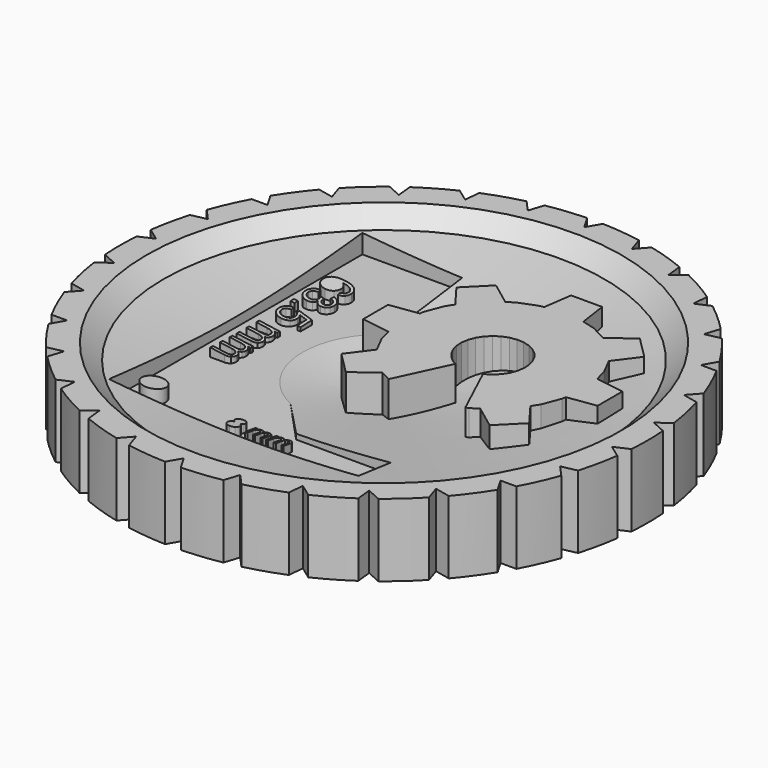
from build123d import *

# Parameters (mm, degrees)
F4_DEPTH        = 64
F4_COPIES_COUNT = 30
F5_R            = 1.080516378
F5_W            = 0.3783217323
F5_H            = 0.3783222047
F6_DEPTH        = 28.3


# Not quite as in the source:
# - ends of sketch curves that miss each other by under 0.0002 mm in the source are joined
# - the dataset's text gives a spline's control points without its knots; the knots are read off the source's solid
# - a pattern or mirror of a feature is missing from the dataset's text; its kind, count and spacing are read off the source's solid


with BuildPart() as f1:
    # F0 (on Front) → F1 (revolve)
    with BuildSketch(Plane.XZ):
        Polygon((-25, 0), (0, 0), (0, 2.5), (-20.8576644046, 5.4197078553), (-22.5, 6.8795619782), (-25, 6.8795619782), align=None)
    revolve(axis=Axis((0, 0, 1.25), (0, 0, -1)))

    # F3 (on offset) → F4 (cut)
    with BuildSketch(Plane.XY.offset(31.8795619782)):
        Polygon((1.4257947543, 26.1719338596), (-1.4257947543, 26.1719338596), (0, 23.702384904), align=None)
    f4 = extrude(amount=-F4_DEPTH, mode=Mode.SUBTRACT)

    # F4_copies: F4 ×30 about axis
    f4_copies_axis = Axis((0, 0, 0), (0, 0, 1))
    for i in range(1, F4_COPIES_COUNT):
        add(f4.rotate(f4_copies_axis, i * 360 / F4_COPIES_COUNT), mode=Mode.SUBTRACT)

    # F5 (on offset) → F6 (cut)
    with BuildSketch(Plane.XY.offset(31.8795619782)):
        Polygon((-14.0490727499, 14.9999975413), (-14.0490727499, -15.0000024587), (9.5729744942, -15.0000024587), (9.5990074076, -11.2204748996), (0.659531817, -11.2204748996), (-4.6002538523, -5.5511835611), (-4.6002538523, 14.9999975413), align=None)
        with Locations((-11.6868680255, -12.6377977343)):
            Circle(F5_R, mode=Mode.SUBTRACT)
        with BuildLine():
            add(Edge.make_bspline(
                [(-3.9348817263, -13.1844435611), (-3.9031511751, -13.150072065), (-3.8372267657, -13.0786621437), (-3.7446949546, -13.0484429311), (-3.6967006239, -13.0327687579)],
                knots=[0, 0, 0, 0, 0.291983, 0.606627, 0.606627, 0.606627, 0.606627], degree=3))
            add(Edge.make_bspline(
                [(-3.6967006239, -13.0327687579), (-3.7361725924, -13.016399624), (-3.8102612538, -12.9856748996), (-3.8633593641, -12.9257958445), (-3.888168183, -12.8978183642)],
                knots=[0, 0, 0, 0, 0.267234, 0.501594, 0.501594, 0.501594, 0.501594], degree=3))
            add(Edge.make_bspline(
                [(-3.888168183, -12.8978183642), (-3.9063288129, -12.8664988366), (-3.9439445609, -12.8016256083), (-3.9482343247, -12.7266662382), (-3.9504529074, -12.6878958445)],
                knots=[0, 0, 0, 0, 0.226571, 0.469298, 0.469298, 0.469298, 0.469298], degree=3))
            add(Edge.make_bspline(
                [(-3.9504529074, -12.6878958445), (-3.9449877105, -12.6288893878), (-3.9340866082, -12.5112010414), (-3.8564971594, -12.4220689154), (-3.8178099153, -12.3776259233)],
                knots=[0, 0, 0, 0, 0.366285, 0.730555, 0.730555, 0.730555, 0.730555], degree=3))
            add(Edge.make_bspline(
                [(-3.8178099153, -12.3776259233), (-3.7682073956, -12.3409834036), (-3.6635744822, -12.2636892303), (-3.533351805, -12.2559652933), (-3.4648629861, -12.2519032461)],
                knots=[0, 0, 0, 0, 0.383224, 0.808383, 0.808383, 0.808383, 0.808383], degree=3))
            add(Edge.make_bspline(
                [(-3.4648629861, -12.2519032461), (-3.3958516476, -12.2561580492), (-3.2641351121, -12.2642783642), (-3.1586659783, -12.3430229311), (-3.108456372, -12.3805097028)],
                knots=[0, 0, 0, 0, 0.428413, 0.817672, 0.817672, 0.817672, 0.817672], degree=3))
            add(Edge.make_bspline(
                [(-3.108456372, -12.3805097028), (-3.0690958995, -12.4256211988), (-2.9905988916, -12.5155876555), (-2.9791927499, -12.6344174193), (-2.9735059783, -12.6936629311)],
                knots=[0, 0, 0, 0, 0.370122, 0.73814, 0.73814, 0.73814, 0.73814], degree=3))
            add(Edge.make_bspline(
                [(-2.9735059783, -12.6936629311), (-2.9757977893, -12.7312045059), (-2.980264246, -12.8043752146), (-3.0172195216, -12.8676057658), (-3.0352143247, -12.8983952146)],
                knots=[0, 0, 0, 0, 0.235128, 0.45828, 0.45828, 0.45828, 0.45828], degree=3))
            add(Edge.make_bspline(
                [(-3.0352143247, -12.8983952146), (-3.0596026712, -12.9261794666), (-3.111556057, -12.9853659233), (-3.1841362145, -13.0163367894), (-3.2226448759, -13.0327687579)],
                knots=[0, 0, 0, 0, 0.231762, 0.493704, 0.493704, 0.493704, 0.493704], degree=3))
            add(Edge.make_bspline(
                [(-3.2226448759, -13.0327687579), (-3.1744984192, -13.0513942697), (-3.0822292853, -13.0870886004), (-3.0168708601, -13.1611423012), (-2.9856170019, -13.1965545847)],
                knots=[0, 0, 0, 0, 0.322391, 0.617832, 0.617832, 0.617832, 0.617832], degree=3))
            add(Edge.make_bspline(
                [(-2.9856170019, -13.1965545847), (-2.9619066082, -13.2368476555), (-2.9129177893, -13.3200983642), (-2.9072338523, -13.4166393091), (-2.9043009389, -13.4664548996)],
                knots=[0, 0, 0, 0, 0.29248, 0.604301, 0.604301, 0.604301, 0.604301], degree=3))
            add(Edge.make_bspline(
                [(-2.9043009389, -13.4664548996), (-2.9105593641, -13.5357232461), (-2.923012435, -13.6735479705), (-3.0129628287, -13.7786542697), (-3.0577058208, -13.8309355296)],
                knots=[0, 0, 0, 0, 0.430093, 0.855761, 0.855761, 0.855761, 0.855761], degree=3))
            add(Edge.make_bspline(
                [(-3.0577058208, -13.8309355296), (-3.1146108601, -13.8739725374), (-3.2337902302, -13.9641076555), (-3.3832870806, -13.9736089154), (-3.4614028287, -13.9785733248)],
                knots=[0, 0, 0, 0, 0.443046, 0.927898, 0.927898, 0.927898, 0.927898], degree=3))
            add(Edge.make_bspline(
                [(-3.4614028287, -13.9785733248), (-3.5395341672, -13.9735753721), (-3.6891316476, -13.9640060807), (-3.8082127499, -13.8735643485), (-3.8650998365, -13.8303586792)],
                knots=[0, 0, 0, 0, 0.484901, 0.928432, 0.928432, 0.928432, 0.928432], degree=3))
            add(Edge.make_bspline(
                [(-3.8650998365, -13.8303586792), (-3.9098418838, -13.7775189941), (-4.0002821987, -13.6707095453), (-4.0123880255, -13.5311868681), (-4.0185047184, -13.460687813)],
                knots=[0, 0, 0, 0, 0.428425, 0.866013, 0.866013, 0.866013, 0.866013], degree=3))
            add(Edge.make_bspline(
                [(-4.0185047184, -13.460687813), (-4.0157031436, -13.4088813563), (-4.0103451909, -13.3097972618), (-3.9592582617, -13.2249355296), (-3.9348817263, -13.1844435611)],
                knots=[0, 0, 0, 0, 0.323778, 0.619255, 0.619255, 0.619255, 0.619255], degree=3))
        make_face(mode=Mode.SUBTRACT)
        with BuildLine():
            Line((-12.5727103877, -2.550036002), (-12.5727103877, -2.2178509626))
            Line((-12.5727103877, -2.2178509626), (-10.6128188916, -2.2178509626))
            Line((-10.6128188916, -2.2178509626), (-10.6128188916, -2.5149714351))
            Line((-10.6128188916, -2.5149714351), (-10.8877941672, -2.5149714351))
            add(Edge.make_bspline(
                [(-10.8877941672, -2.5149714351), (-10.8420387342, -2.5484750571), (-10.7497648759, -2.6160407264), (-10.6875514901, -2.7120293878), (-10.6561875531, -2.7604205689)],
                knots=[0, 0, 0, 0, 0.356855, 0.719659, 0.719659, 0.719659, 0.719659], degree=3))
            add(Edge.make_bspline(
                [(-10.6561875531, -2.7604205689), (-10.6306251909, -2.8140846634), (-10.5780789601, -2.9243975906), (-10.5717685144, -3.0465068651), (-10.5685275777, -3.1092133202)],
                knots=[0, 0, 0, 0, 0.373568, 0.767905, 0.767905, 0.767905, 0.767905], degree=3))
            add(Edge.make_bspline(
                [(-10.5685275777, -3.1092133202), (-10.5710919625, -3.1765810414), (-10.5758792066, -3.3023174193), (-10.6326165294, -3.414319939), (-10.6589555846, -3.4663134823)],
                knots=[0, 0, 0, 0, 0.422154, 0.787929, 0.787929, 0.787929, 0.787929], degree=3))
            add(Edge.make_bspline(
                [(-10.6589555846, -3.4663134823), (-10.6923566869, -3.5094260807), (-10.7598154864, -3.5964996549), (-10.8608004877, -3.6405935115), (-10.9117847502, -3.6628553372)],
                knots=[0, 0, 0, 0, 0.340443, 0.687583, 0.687583, 0.687583, 0.687583], degree=3))
            add(Edge.make_bspline(
                [(-10.9117847502, -3.6628553372), (-10.8116985767, -3.7441177343), (-10.6176892853, -3.9016366319), (-10.5845640885, -4.1486093878), (-10.5685275531, -4.2681714351)],
                knots=[0, 0, 0, 0, 0.785976, 1.523536, 1.523536, 1.523536, 1.523536], degree=3))
            add(Edge.make_bspline(
                [(-10.5685275531, -4.2681714351), (-10.5730776318, -4.357499624), (-10.5815631436, -4.5240865532), (-10.6829740098, -4.6556193091), (-10.7300064507, -4.7166213563)],
                knots=[0, 0, 0, 0, 0.552547, 1.030438, 1.030438, 1.030438, 1.030438], degree=3))
            add(Edge.make_bspline(
                [(-10.7300064507, -4.7166213563), (-10.796196372, -4.7622308051), (-10.9449448759, -4.8647297028), (-11.1265606239, -4.8703607264), (-11.2273610964, -4.8734863957)],
                knots=[0, 0, 0, 0, 0.50044, 1.124636, 1.124636, 1.124636, 1.124636], degree=3))
            Line((-11.2273610964, -4.8734863957), (-12.5727103877, -4.8734863957))
            Line((-12.5727103877, -4.8734863957), (-12.5727103877, -4.5431462382))
            Line((-12.5727103877, -4.5431462382), (-11.3380894428, -4.5431462382))
            add(Edge.make_bspline(
                [(-11.3380894428, -4.5431462382), (-11.2806151121, -4.5431325374), (-11.1835884979, -4.5431098603), (-11.0894810964, -4.5201926949), (-11.0511184192, -4.5108506477)],
                knots=[0, 0, 0, 0, 0.363195, 0.613139, 0.613139, 0.613139, 0.613139], degree=3))
            add(Edge.make_bspline(
                [(-11.0511184192, -4.5108506477), (-11.0231555846, -4.4976279705), (-10.9661244035, -4.4706600965), (-10.9289088129, -4.4196586792), (-10.9099398365, -4.3936635611)],
                knots=[0, 0, 0, 0, 0.193139, 0.393917, 0.393917, 0.393917, 0.393917], degree=3))
            add(Edge.make_bspline(
                [(-10.9099398365, -4.3936635611), (-10.8943355846, -4.3635147422), (-10.8620038358, -4.3010471353), (-10.8583247684, -4.230732391), (-10.8564213289, -4.1943539714)],
                knots=[0, 0, 0, 0, 0.212991, 0.441316, 0.441316, 0.441316, 0.441316], degree=3))
            add(Edge.make_bspline(
                [(-10.8564213289, -4.1943539714), (-10.8617229861, -4.1288065532), (-10.8721384192, -4.0000474981), (-10.95381212, -3.9001418288), (-10.9939086554, -3.8510939548)],
                knots=[0, 0, 0, 0, 0.406947, 0.799408, 0.799408, 0.799408, 0.799408], degree=3))
            add(Edge.make_bspline(
                [(-10.9939086554, -3.8510939548), (-11.051635742, -3.8114150571), (-11.1832118301, -3.7209748331), (-11.343877466, -3.7168465615), (-11.4340535249, -3.7145297152)],
                knots=[0, 0, 0, 0, 0.436121, 0.994043, 0.994043, 0.994043, 0.994043], degree=3))
            Line((-11.4340535249, -3.7145297152), (-12.5727103877, -3.7145297028))
            Line((-12.5727103877, -3.7145297028), (-12.5727103877, -3.3823446634))
            Line((-12.5727103877, -3.3823446634), (-11.2993346397, -3.3823446634))
            add(Edge.make_bspline(
                [(-11.2993346397, -3.3823446634), (-11.2332944822, -3.381036002), (-11.1159987342, -3.3787115925), (-11.0124136948, -3.3247314351), (-10.9671496003, -3.3011434036)],
                knots=[0, 0, 0, 0, 0.412401, 0.732475, 0.732475, 0.732475, 0.732475], degree=3))
            add(Edge.make_bspline(
                [(-10.9671496003, -3.3011434036), (-10.9349173168, -3.2674758445), (-10.8643549546, -3.1937708051), (-10.8592138523, -3.0911434036), (-10.8564212538, -3.0353948996)],
                knots=[0, 0, 0, 0, 0.286757, 0.627767, 0.627767, 0.627767, 0.627767], degree=3))
            add(Edge.make_bspline(
                [(-10.8564212538, -3.0353948996), (-10.8594925924, -2.9895345847), (-10.8656329074, -2.8978470256), (-10.9087096003, -2.8166769469), (-10.9302401515, -2.7761065532)],
                knots=[0, 0, 0, 0, 0.288303, 0.576397, 0.576397, 0.576397, 0.576397], degree=3))
            add(Edge.make_bspline(
                [(-10.9302401515, -2.7761065532), (-10.9581902302, -2.7389741122), (-11.0153403701, -2.6630492008), (-11.1019220644, -2.623673615), (-11.1461598713, -2.6035552562)],
                knots=[0, 0, 0, 0, 0.290214, 0.593409, 0.593409, 0.593409, 0.593409], degree=3))
            add(Edge.make_bspline(
                [(-11.1461598713, -2.6035552562), (-11.2036776318, -2.5880235611), (-11.3376221987, -2.5518539548), (-11.476571805, -2.5506964744), (-11.5558549546, -2.550036002)],
                knots=[0, 0, 0, 0, 0.376888, 0.87769, 0.87769, 0.87769, 0.87769], degree=3))
            Line((-11.5558549546, -2.550036002), (-12.5727103877, -2.550036002))
        make_face(mode=Mode.SUBTRACT)
        with BuildLine():
            Line((-12.5727103877, 0.5983406909), (-12.5727103877, 0.9305257303))
            Line((-12.5727103877, 0.9305257303), (-10.6128188916, 0.9305257303))
            Line((-10.6128188916, 0.9305257303), (-10.6128188916, 0.633404313))
            Line((-10.6128188916, 0.633404313), (-10.8877941672, 0.633404313))
            add(Edge.make_bspline(
                [(-10.8877941672, 0.633404313), (-10.8420387342, 0.5999011634), (-10.7497648759, 0.5323354941), (-10.6875514901, 0.4363477775), (-10.6561875531, 0.3879570689)],
                knots=[0, 0, 0, 0, 0.356855, 0.719659, 0.719659, 0.719659, 0.719659], degree=3))
            add(Edge.make_bspline(
                [(-10.6561875531, 0.3879570689), (-10.6306251909, 0.3342920295), (-10.5780793641, 0.2239784862), (-10.5717684979, 0.1018690374), (-10.5685275531, 0.0391628956)],
                knots=[0, 0, 0, 0, 0.373568, 0.767906, 0.767906, 0.767906, 0.767906], degree=3))
            add(Edge.make_bspline(
                [(-10.5685275531, 0.0391628956), (-10.571092435, -0.028203876), (-10.5758792066, -0.153940254), (-10.6326165294, -0.2659427737), (-10.6589555846, -0.3179367894)],
                knots=[0, 0, 0, 0, 0.422154, 0.787929, 0.787929, 0.787929, 0.787929], degree=3))
            add(Edge.make_bspline(
                [(-10.6589555846, -0.3179367894), (-10.6923562145, -0.3610498603), (-10.7598151121, -0.4481245059), (-10.8608007814, -0.4922178918), (-10.9117851909, -0.5144788366)],
                knots=[0, 0, 0, 0, 0.340443, 0.687584, 0.687584, 0.687584, 0.687584], degree=3))
            add(Edge.make_bspline(
                [(-10.9117851909, -0.5144788366), (-10.8116985767, -0.5957415138), (-10.6176897578, -0.7532604114), (-10.5845640885, -1.0002331674), (-10.5685275531, -1.1197947422)],
                knots=[0, 0, 0, 0, 0.785976, 1.523536, 1.523536, 1.523536, 1.523536], degree=3))
            add(Edge.make_bspline(
                [(-10.5685275531, -1.1197947422), (-10.5730776318, -1.2091234036), (-10.5815626712, -1.3757108051), (-10.6829740098, -1.5072430886), (-10.7300064507, -1.5682446634)],
                knots=[0, 0, 0, 0, 0.552547, 1.030438, 1.030438, 1.030438, 1.030438], degree=3))
            add(Edge.make_bspline(
                [(-10.7300064507, -1.5682446634), (-10.796196372, -1.6138541122), (-10.9449448759, -1.7163530099), (-11.1265606239, -1.7219840335), (-11.2273610964, -1.7251097028)],
                knots=[0, 0, 0, 0, 0.50044, 1.124636, 1.124636, 1.124636, 1.124636], degree=3))
            Line((-11.2273610964, -1.7251097028), (-12.5727103877, -1.7251097028))
            Line((-12.5727103877, -1.7251097028), (-12.5727103877, -1.3947695453))
            Line((-12.5727103877, -1.3947695453), (-11.3380894428, -1.3947695453))
            add(Edge.make_bspline(
                [(-11.3380894428, -1.3947695453), (-11.2806151121, -1.3947558445), (-11.1835884979, -1.3947331674), (-11.0894810964, -1.371816002), (-11.0511184192, -1.3624739548)],
                knots=[0, 0, 0, 0, 0.363195, 0.613139, 0.613139, 0.613139, 0.613139], degree=3))
            add(Edge.make_bspline(
                [(-11.0511184192, -1.3624739548), (-11.0231555846, -1.3492512776), (-10.9661244035, -1.3222834036), (-10.9289088129, -1.2712819863), (-10.9099398365, -1.2452868681)],
                knots=[0, 0, 0, 0, 0.193139, 0.393917, 0.393917, 0.393917, 0.393917], degree=3))
            add(Edge.make_bspline(
                [(-10.9099398365, -1.2452868681), (-10.8943355846, -1.2151380492), (-10.8620031436, -1.1526704902), (-10.8583247184, -1.0823547422), (-10.8564212538, -1.0459748996)],
                knots=[0, 0, 0, 0, 0.212991, 0.441319, 0.441319, 0.441319, 0.441319], degree=3))
            add(Edge.make_bspline(
                [(-10.8564212538, -1.0459748996), (-10.8617229861, -0.9804289154), (-10.8721379468, -0.8516698603), (-10.95381212, -0.7517646634), (-10.9939086554, -0.7027172618)],
                knots=[0, 0, 0, 0, 0.406947, 0.799408, 0.799408, 0.799408, 0.799408], degree=3))
            add(Edge.make_bspline(
                [(-10.9939086554, -0.7027172618), (-11.051635742, -0.6630378918), (-11.1832114901, -0.5725966319), (-11.3438777893, -0.5684689154), (-11.4340540098, -0.566152065)],
                knots=[0, 0, 0, 0, 0.436121, 0.994044, 0.994044, 0.994044, 0.994044], degree=3))
            Line((-11.4340540098, -0.566152065), (-12.5727103877, -0.566152065))
            Line((-12.5727103877, -0.566152065), (-12.5727103877, -0.2339670256))
            Line((-12.5727103877, -0.2339670256), (-11.2993346397, -0.2339670256))
            add(Edge.make_bspline(
                [(-11.2993346397, -0.2339670256), (-11.2332944822, -0.2326588366), (-11.1159987342, -0.2303348996), (-11.0124136948, -0.1763547422), (-10.9671496003, -0.1527667107)],
                knots=[0, 0, 0, 0, 0.412401, 0.732475, 0.732475, 0.732475, 0.732475], degree=3))
            add(Edge.make_bspline(
                [(-10.9671496003, -0.1527667107), (-10.9349173168, -0.119099624), (-10.8643544822, -0.0453950571), (-10.8592138523, 0.0572328169), (-10.8564212538, 0.1129817933)],
                knots=[0, 0, 0, 0, 0.286757, 0.627767, 0.627767, 0.627767, 0.627767], degree=3))
            add(Edge.make_bspline(
                [(-10.8564212538, 0.1129817933), (-10.8594925924, 0.1588421082), (-10.8656329074, 0.2505296673), (-10.9087096003, 0.331699746), (-10.9302401515, 0.3722701397)],
                knots=[0, 0, 0, 0, 0.288303, 0.576397, 0.576397, 0.576397, 0.576397], degree=3))
            add(Edge.make_bspline(
                [(-10.9302401515, 0.3722701397), (-10.9581902302, 0.4094021082), (-11.0153404664, 0.48532762), (-11.1019223562, 0.5247032106), (-11.146160309, 0.5448221082)],
                knots=[0, 0, 0, 0, 0.290214, 0.59341, 0.59341, 0.59341, 0.59341], degree=3))
            add(Edge.make_bspline(
                [(-11.146160309, 0.5448221082), (-11.2036776318, 0.5603536043), (-11.3376221987, 0.5965232106), (-11.476571805, 0.5976802185), (-11.5558549546, 0.5983406909)],
                knots=[0, 0, 0, 0, 0.376888, 0.87769, 0.87769, 0.87769, 0.87769], degree=3))
            Line((-11.5558549546, 0.5983406909), (-12.5727103877, 0.5983406909))
        make_face(mode=Mode.SUBTRACT)
        with BuildLine():
            Line((-1.7808694428, -13.9497378918), (-1.9884850334, -13.9497378918))
            Line((-1.9884850334, -13.9497378918), (-1.9884850334, -12.7248052933))
            Line((-1.9884850334, -12.7248052933), (-1.8027845609, -12.7248052933))
            Line((-1.8027845609, -12.7248052933), (-1.8027845609, -12.8966651359))
            add(Edge.make_bspline(
                [(-1.8027845609, -12.8966651359), (-1.7818450334, -12.868067813), (-1.7396168444, -12.8103969469), (-1.679623931, -12.7715131674), (-1.649379679, -12.7519106477)],
                knots=[0, 0, 0, 0, 0.223034, 0.449787, 0.449787, 0.449787, 0.449787], degree=3))
            add(Edge.make_bspline(
                [(-1.649379679, -12.7519106477), (-1.6158392066, -12.7359345847), (-1.5468935373, -12.7030933248), (-1.4705749546, -12.6991489154), (-1.4313831436, -12.6971235611)],
                knots=[0, 0, 0, 0, 0.233479, 0.479942, 0.479942, 0.479942, 0.479942], degree=3))
            add(Edge.make_bspline(
                [(-1.4313831436, -12.6971235611), (-1.3892792066, -12.6987265532), (-1.3106938523, -12.7017180492), (-1.2406927499, -12.7371789941), (-1.208196372, -12.7536411988)],
                knots=[0, 0, 0, 0, 0.263846, 0.492455, 0.492455, 0.492455, 0.492455], degree=3))
            add(Edge.make_bspline(
                [(-1.208196372, -12.7536411988), (-1.1812507027, -12.7745164744), (-1.1268292853, -12.8166780492), (-1.0992708601, -12.8797942697), (-1.0853570019, -12.9116594666)],
                knots=[0, 0, 0, 0, 0.212777, 0.42974, 0.42974, 0.42974, 0.42974], degree=3))
            add(Edge.make_bspline(
                [(-1.0853570019, -12.9116594666), (-1.034568183, -12.8491049784), (-0.9361190491, -12.7278497028), (-0.7817617263, -12.7071459233), (-0.7070352696, -12.6971235611)],
                knots=[0, 0, 0, 0, 0.491234, 0.952209, 0.952209, 0.952209, 0.952209], degree=3))
            add(Edge.make_bspline(
                [(-0.7070352696, -12.6971235611), (-0.6512050334, -12.6999671831), (-0.5470880255, -12.7052703327), (-0.4648804664, -12.7686525374), (-0.4267540098, -12.798047813)],
                knots=[0, 0, 0, 0, 0.345341, 0.644024, 0.644024, 0.644024, 0.644024], degree=3))
            add(Edge.make_bspline(
                [(-0.4267540098, -12.798047813), (-0.398247868, -12.8394166319), (-0.3341862932, -12.9323845059), (-0.3306670806, -13.0458941122), (-0.3287135373, -13.1088945847)],
                knots=[0, 0, 0, 0, 0.312775, 0.702897, 0.702897, 0.702897, 0.702897], degree=3))
            Line((-0.3287135373, -13.1088945847), (-0.3287135373, -13.9497378918))
            Line((-0.3287135373, -13.9497378918), (-0.5351754271, -13.9497378918))
            Line((-0.5351754271, -13.9497378918), (-0.5351754271, -13.178099624))
            add(Edge.make_bspline(
                [(-0.5351754271, -13.178099624), (-0.535183931, -13.1421780492), (-0.5351985767, -13.0815364744), (-0.5495215688, -13.0227194666), (-0.5553604664, -12.9987426162)],
                knots=[0, 0, 0, 0, 0.226997, 0.383212, 0.383212, 0.383212, 0.383212], degree=3))
            add(Edge.make_bspline(
                [(-0.5553604664, -12.9987426162), (-0.5636244035, -12.9812660807), (-0.5804792066, -12.9456213563), (-0.6123552696, -12.9223616713), (-0.6286025137, -12.9105062382)],
                knots=[0, 0, 0, 0, 0.120712, 0.246199, 0.246199, 0.246199, 0.246199], degree=3))
            add(Edge.make_bspline(
                [(-0.6286025137, -12.9105062382), (-0.6474453483, -12.9007531674), (-0.686487868, -12.8805459233), (-0.7304347972, -12.8782465532), (-0.7531719625, -12.8770569469)],
                knots=[0, 0, 0, 0, 0.13312, 0.275823, 0.275823, 0.275823, 0.275823], degree=3))
            add(Edge.make_bspline(
                [(-0.7531719625, -12.8770569469), (-0.7941382617, -12.8803706477), (-0.8746129074, -12.886879939), (-0.9370535373, -12.9379262382), (-0.9677083405, -12.9629868681)],
                knots=[0, 0, 0, 0, 0.254342, 0.49963, 0.49963, 0.49963, 0.49963], degree=3))
            add(Edge.make_bspline(
                [(-0.9677083405, -12.9629868681), (-0.9925077105, -12.9990662382), (-1.0490329074, -13.0813011988), (-1.0516133798, -13.1817171044), (-1.0530614113, -13.2380774193)],
                knots=[0, 0, 0, 0, 0.272575, 0.621277, 0.621277, 0.621277, 0.621277], degree=3))
            Line((-1.0530614113, -13.2380774193), (-1.0530614113, -13.9497378918))
            Line((-1.0530614113, -13.9497378918), (-1.2606770019, -13.9497378918))
            Line((-1.2606770019, -13.9497378918), (-1.2606770019, -13.1538775768))
            add(Edge.make_bspline(
                [(-1.2606770019, -13.1538775768), (-1.2614947972, -13.1126027737), (-1.2629470806, -13.0392926949), (-1.2966850334, -12.9745522225), (-1.3114275531, -12.9462619863)],
                knots=[0, 0, 0, 0, 0.257751, 0.457797, 0.457797, 0.457797, 0.457797], degree=3))
            add(Edge.make_bspline(
                [(-1.3114275531, -12.9462619863), (-1.3324696003, -12.9261171044), (-1.3785349546, -12.8820152146), (-1.4426773168, -12.8788021437), (-1.4775198365, -12.8770569469)],
                knots=[0, 0, 0, 0, 0.179223, 0.392354, 0.392354, 0.392354, 0.392354], degree=3))
            add(Edge.make_bspline(
                [(-1.4775198365, -12.8770569469), (-1.5061828287, -12.8789764744), (-1.5634875531, -12.8828141122), (-1.6142192066, -12.9097371044), (-1.6395755846, -12.9231936398)],
                knots=[0, 0, 0, 0, 0.180189, 0.360249, 0.360249, 0.360249, 0.360249], degree=3))
            add(Edge.make_bspline(
                [(-1.6395755846, -12.9231936398), (-1.6627833011, -12.9406626162), (-1.7102366869, -12.9763815138), (-1.7348461357, -13.0304953721), (-1.7474201515, -13.0581440335)],
                knots=[0, 0, 0, 0, 0.181384, 0.370881, 0.370881, 0.370881, 0.370881], degree=3))
            add(Edge.make_bspline(
                [(-1.7474201515, -13.0581440335), (-1.757127868, -13.094092065), (-1.7797336948, -13.1778076555), (-1.7804570019, -13.2646512776), (-1.7808694428, -13.3142032461)],
                knots=[0, 0, 0, 0, 0.235555, 0.548556, 0.548556, 0.548556, 0.548556], degree=3))
            Line((-1.7808694428, -13.3142032461), (-1.7808694428, -13.9497378918))
        make_face(mode=Mode.SUBTRACT)
        with BuildLine():
            Line((0.1868655178, -13.9497378918), (-0.0207500727, -13.9497378918))
            Line((-0.0207500727, -13.9497378918), (-0.0207500727, -12.7248052933))
            Line((-0.0207500727, -12.7248052933), (0.1649503997, -12.7248052933))
            Line((0.1649503997, -12.7248052933), (0.1649503997, -12.8966651359))
            add(Edge.make_bspline(
                [(0.1649503997, -12.8966651359), (0.1858899273, -12.868067813), (0.2281185887, -12.8103969469), (0.2881110296, -12.7715131674), (0.3183552816, -12.7519106477)],
                knots=[0, 0, 0, 0, 0.223034, 0.449787, 0.449787, 0.449787, 0.449787], degree=3))
            add(Edge.make_bspline(
                [(0.3183552816, -12.7519106477), (0.351895754, -12.7359345847), (0.4208414233, -12.7030933248), (0.497160006, -12.6991489154), (0.536351817, -12.6971235611)],
                knots=[0, 0, 0, 0, 0.233479, 0.479942, 0.479942, 0.479942, 0.479942], degree=3))
            add(Edge.make_bspline(
                [(0.536351817, -12.6971235611), (0.578455754, -12.6987265532), (0.6570411084, -12.7017180492), (0.7270422107, -12.7371789941), (0.7595385887, -12.7536411988)],
                knots=[0, 0, 0, 0, 0.263846, 0.492455, 0.492455, 0.492455, 0.492455], degree=3))
            add(Edge.make_bspline(
                [(0.7595385887, -12.7536411988), (0.786484258, -12.7745164744), (0.8409056753, -12.8166780492), (0.8684641005, -12.8797942697), (0.8823779587, -12.9116594666)],
                knots=[0, 0, 0, 0, 0.212777, 0.42974, 0.42974, 0.42974, 0.42974], degree=3))
            add(Edge.make_bspline(
                [(0.8823779587, -12.9116594666), (0.9331667776, -12.8491049784), (1.0316159115, -12.7278497028), (1.1859732343, -12.7071459233), (1.260699691, -12.6971235611)],
                knots=[0, 0, 0, 0, 0.491234, 0.952209, 0.952209, 0.952209, 0.952209], degree=3))
            add(Edge.make_bspline(
                [(1.260699691, -12.6971235611), (1.3165299273, -12.6999671831), (1.4206469351, -12.7052703327), (1.5028549666, -12.7686525374), (1.5409809509, -12.798047813)],
                knots=[0, 0, 0, 0, 0.345341, 0.644024, 0.644024, 0.644024, 0.644024], degree=3))
            add(Edge.make_bspline(
                [(1.5409809509, -12.798047813), (1.5694870926, -12.8394166319), (1.6335486674, -12.9323845059), (1.6370683524, -13.0458941122), (1.6390214233, -13.1088945847)],
                knots=[0, 0, 0, 0, 0.312775, 0.702897, 0.702897, 0.702897, 0.702897], degree=3))
            Line((1.6390214233, -13.1088945847), (1.6390214233, -13.9497378918))
            Line((1.6390214233, -13.9497378918), (1.4325595336, -13.9497378918))
            Line((1.4325595336, -13.9497378918), (1.4325595336, -13.178099624))
            add(Edge.make_bspline(
                [(1.4325595336, -13.178099624), (1.4325510296, -13.1421780492), (1.4325363839, -13.0815364744), (1.4182133918, -13.0227194666), (1.4123744942, -12.9987426162)],
                knots=[0, 0, 0, 0, 0.226997, 0.383212, 0.383212, 0.383212, 0.383212], degree=3))
            add(Edge.make_bspline(
                [(1.4123744942, -12.9987426162), (1.4041105572, -12.9812660807), (1.387255754, -12.9456213563), (1.355379691, -12.9223616713), (1.3391324469, -12.9105062382)],
                knots=[0, 0, 0, 0, 0.120712, 0.246199, 0.246199, 0.246199, 0.246199], degree=3))
            add(Edge.make_bspline(
                [(1.3391324469, -12.9105062382), (1.3202896123, -12.9007531674), (1.2812470926, -12.8805459233), (1.2373001635, -12.8782465532), (1.2145629981, -12.8770569469)],
                knots=[0, 0, 0, 0, 0.13312, 0.275823, 0.275823, 0.275823, 0.275823], degree=3))
            add(Edge.make_bspline(
                [(1.2145629981, -12.8770569469), (1.1735966989, -12.8803706477), (1.0931220532, -12.886879939), (1.0306814233, -12.9379262382), (1.0000266202, -12.9629868681)],
                knots=[0, 0, 0, 0, 0.254342, 0.49963, 0.49963, 0.49963, 0.49963], degree=3))
            add(Edge.make_bspline(
                [(1.0000266202, -12.9629868681), (0.9752272501, -12.9990662382), (0.9187020532, -13.0813011988), (0.9161215808, -13.1817171044), (0.9146735493, -13.2380774193)],
                knots=[0, 0, 0, 0, 0.272575, 0.621277, 0.621277, 0.621277, 0.621277], degree=3))
            Line((0.9146735493, -13.2380774193), (0.9146735493, -13.9497378918))
            Line((0.9146735493, -13.9497378918), (0.7070579587, -13.9497378918))
            Line((0.7070579587, -13.9497378918), (0.7070579587, -13.1538775768))
            add(Edge.make_bspline(
                [(0.7070579587, -13.1538775768), (0.7062401635, -13.1126027737), (0.70478788, -13.0392926949), (0.6710499273, -12.9745522225), (0.6563074076, -12.9462619863)],
                knots=[0, 0, 0, 0, 0.257751, 0.457797, 0.457797, 0.457797, 0.457797], degree=3))
            add(Edge.make_bspline(
                [(0.6563074076, -12.9462619863), (0.6352653603, -12.9261171044), (0.589200006, -12.8820152146), (0.5250576438, -12.8788021437), (0.4902151241, -12.8770569469)],
                knots=[0, 0, 0, 0, 0.179223, 0.392354, 0.392354, 0.392354, 0.392354], degree=3))
            add(Edge.make_bspline(
                [(0.4902151241, -12.8770569469), (0.461552132, -12.8789764744), (0.4042474076, -12.8828141122), (0.353515754, -12.9097371044), (0.3281593761, -12.9231936398)],
                knots=[0, 0, 0, 0, 0.180189, 0.360249, 0.360249, 0.360249, 0.360249], degree=3))
            add(Edge.make_bspline(
                [(0.3281593761, -12.9231936398), (0.3049516595, -12.9406626162), (0.2574987462, -12.9763815138), (0.2328888249, -13.0304953721), (0.2203148091, -13.0581440335)],
                knots=[0, 0, 0, 0, 0.181384, 0.370881, 0.370881, 0.370881, 0.370881], degree=3))
            add(Edge.make_bspline(
                [(0.2203148091, -13.0581440335), (0.2106070926, -13.094092065), (0.1880012658, -13.1778076555), (0.1872779587, -13.2646512776), (0.1868655178, -13.3142032461)],
                knots=[0, 0, 0, 0, 0.235555, 0.548556, 0.548556, 0.548556, 0.548556], degree=3))
            Line((0.1868655178, -13.3142032461), (0.1868655178, -13.9497378918))
        make_face(mode=Mode.SUBTRACT)
        with BuildLine():
            add(Edge.make_bspline(
                [(-12.4121546397, 3.9081948641), (-12.3362059783, 3.9777972263), (-12.180175742, 4.1207895098), (-11.9712694428, 4.1565249429), (-11.8640489704, 4.1748660452)],
                knots=[0, 0, 0, 0, 0.639963, 1.31476, 1.31476, 1.31476, 1.31476], degree=3))
            Line((-11.8640489704, 4.1748660452), (-11.8345214113, 3.826071872))
            add(Edge.make_bspline(
                [(-11.8345214113, 3.826071872), (-11.9120253483, 3.8110756515), (-12.0553804664, 3.7833376988), (-12.1664409389, 3.689324313), (-12.2174570019, 3.6461380137)],
                knots=[0, 0, 0, 0, 0.491428, 0.908973, 0.908973, 0.908973, 0.908973], degree=3))
            add(Edge.make_bspline(
                [(-12.2174570019, 3.6461380137), (-12.2548648759, 3.5962610059), (-12.3306023562, 3.4952781712), (-12.3406384192, 3.3693688799), (-12.3457176318, 3.3056484075)],
                knots=[0, 0, 0, 0, 0.387412, 0.784371, 0.784371, 0.784371, 0.784371], degree=3))
            add(Edge.make_bspline(
                [(-12.3457176318, 3.3056484075), (-12.337984246, 3.2285734468), (-12.3224154271, 3.0733973838), (-12.2176100727, 2.9578165964), (-12.1648610964, 2.8996444704)],
                knots=[0, 0, 0, 0, 0.47842, 0.963208, 0.963208, 0.963208, 0.963208], degree=3))
            add(Edge.make_bspline(
                [(-12.1648610964, 2.8996444704), (-12.0971962145, 2.8512395886), (-11.9540844035, 2.7488625807), (-11.7779140098, 2.7388369114), (-11.6850382617, 2.7335517145)],
                knots=[0, 0, 0, 0, 0.517519, 1.094564, 1.094564, 1.094564, 1.094564], degree=3))
            add(Edge.make_bspline(
                [(-11.6850382617, 2.7335517145), (-11.5971944822, 2.7384523445), (-11.4314607814, 2.7476980137), (-11.2988919625, 2.8466706122), (-11.2365883405, 2.8931852578)],
                knots=[0, 0, 0, 0, 0.544676, 1.027636, 1.027636, 1.027636, 1.027636], degree=3))
            add(Edge.make_bspline(
                [(-11.2365883405, 2.8931852578), (-11.1886984192, 2.9518846279), (-11.0895543247, 3.0734058878), (-11.0782072381, 3.2301528169), (-11.0723414113, 3.3111849429)],
                knots=[0, 0, 0, 0, 0.469248, 0.971455, 0.971455, 0.971455, 0.971455], degree=3))
            add(Edge.make_bspline(
                [(-11.0723414113, 3.3111849429), (-11.0751179468, 3.3629285649), (-11.0805581042, 3.4643077775), (-11.1239787342, 3.5560208484), (-11.1452376318, 3.600923998)],
                knots=[0, 0, 0, 0, 0.325535, 0.637808, 0.637808, 0.637808, 0.637808], degree=3))
            add(Edge.make_bspline(
                [(-11.1452376318, 3.600923998), (-11.1709540098, 3.64142825), (-11.2214069231, 3.7208942342), (-11.2972251909, 3.7766091949), (-11.3343987342, 3.8039257303)],
                knots=[0, 0, 0, 0, 0.301697, 0.591905, 0.591905, 0.591905, 0.591905], degree=3))
            Line((-11.3343987342, 3.8039257303), (-11.2937981042, 4.1158104547))
            Line((-11.2937981042, 4.1158104547), (-9.9041574743, 3.8537540767))
            Line((-9.9041574743, 3.8537540767), (-9.9041574743, 2.5084047854))
            Line((-9.9041574743, 2.5084047854), (-10.2215787342, 2.5084047854))
            Line((-10.2215787342, 2.5084047854), (-10.2215787342, 3.5880060452))
            Line((-10.2215787342, 3.5880060452), (-10.9486946397, 3.7337980137))
            add(Edge.make_bspline(
                [(-10.9486946397, 3.7337980137), (-10.8991861357, 3.6529095098), (-10.80285212, 3.4955172263), (-10.7867418838, 3.3118685649), (-10.7789111751, 3.2226022657)],
                knots=[0, 0, 0, 0, 0.593102, 1.154054, 1.154054, 1.154054, 1.154054], degree=3))
            add(Edge.make_bspline(
                [(-10.7789111751, 3.2226022657), (-10.7888555846, 3.1093874626), (-10.8086088129, 2.8844970689), (-10.9527713326, 2.7108825807), (-11.0243593641, 2.6246691949)],
                knots=[0, 0, 0, 0, 0.703499, 1.39744, 1.39744, 1.39744, 1.39744], degree=3))
            add(Edge.make_bspline(
                [(-11.0243593641, 2.6246691949), (-11.1138793641, 2.5536367539), (-11.2985688129, 2.4070898248), (-11.5341283405, 2.389916124), (-11.6555107027, 2.3810663602)],
                knots=[0, 0, 0, 0, 0.708583, 1.461882, 1.461882, 1.461882, 1.461882], degree=3))
            add(Edge.make_bspline(
                [(-11.6555107027, 2.3810663602), (-11.7728990491, 2.3892943917), (-12.0033325924, 2.4054462027), (-12.1958891279, 2.5327090374), (-12.2903532224, 2.5951416358)],
                knots=[0, 0, 0, 0, 0.73341, 1.439689, 1.439689, 1.439689, 1.439689], degree=3))
            add(Edge.make_bspline(
                [(-12.2903532224, 2.5951416358), (-12.386152435, 2.691312187), (-12.5818469231, 2.8877654153), (-12.6063429861, 3.1644235256), (-12.6188475531, 3.3056484075)],
                knots=[0, 0, 0, 0, 0.834401, 1.704481, 1.704481, 1.704481, 1.704481], degree=3))
            add(Edge.make_bspline(
                [(-12.6188475531, 3.3056484075), (-12.6119513326, 3.421020376), (-12.5987702302, 3.6415284075), (-12.4724045609, 3.822100061), (-12.4121546397, 3.9081948641)],
                knots=[0, 0, 0, 0, 0.717854, 1.372017, 1.372017, 1.372017, 1.372017], degree=3))
        make_face(mode=Mode.SUBTRACT)
        with Locations((-12.3835495216, 4.8493860452)):
            Rectangle(F5_W, F5_H, mode=Mode.SUBTRACT)
        with BuildLine():
            add(Edge.make_bspline(
                [(-12.4084634586, 7.0565715571), (-12.3314593641, 7.1266789586), (-12.1744700727, 7.2696084075), (-11.9651565294, 7.3063619508), (-11.8585129074, 7.32508762)],
                knots=[0, 0, 0, 0, 0.647177, 1.319403, 1.319403, 1.319403, 1.319403], degree=3))
            Line((-11.8585129074, 7.32508762), (-11.8142210964, 6.9929025807))
            add(Edge.make_bspline(
                [(-11.8142210964, 6.9929025807), (-11.8985073956, 6.9737583287), (-12.0494914901, 6.9394647854), (-12.1685522775, 6.8414871476), (-12.221148183, 6.7982054153)],
                knots=[0, 0, 0, 0, 0.539552, 0.966513, 0.966513, 0.966513, 0.966513], degree=3))
            add(Edge.make_bspline(
                [(-12.221148183, 6.7982054153), (-12.2574779468, 6.7493266752), (-12.3314130649, 6.6498528169), (-12.3408949546, 6.526163998), (-12.3457176318, 6.463251872)],
                knots=[0, 0, 0, 0, 0.378519, 0.770334, 0.770334, 0.770334, 0.770334], degree=3))
            add(Edge.make_bspline(
                [(-12.3457176318, 6.463251872), (-12.3391284979, 6.3883416358), (-12.3260352696, 6.23948825), (-12.2306825137, 6.1245126594), (-12.1833155846, 6.0673983287)],
                knots=[0, 0, 0, 0, 0.465521, 0.925031, 0.925031, 0.925031, 0.925031], degree=3))
            add(Edge.make_bspline(
                [(-12.1833155846, 6.0673983287), (-12.1254434586, 6.0203025807), (-12.0081699153, 5.9248671476), (-11.8573804664, 5.9122898248), (-11.7810028287, 5.9059194311)],
                knots=[0, 0, 0, 0, 0.46234, 0.936894, 0.936894, 0.936894, 0.936894], degree=3))
            add(Edge.make_bspline(
                [(-11.7810028287, 5.9059194311), (-11.7086716476, 5.9115513996), (-11.567279994, 5.9225602185), (-11.4573146397, 6.0118099823), (-11.4036037735, 6.0554025807)],
                knots=[0, 0, 0, 0, 0.448919, 0.877538, 0.877538, 0.877538, 0.877538], degree=3))
            add(Edge.make_bspline(
                [(-11.4036037735, 6.0554025807), (-11.3602814113, 6.1095438405), (-11.2713840885, 6.2206416358), (-11.2605812538, 6.3627273051), (-11.2550433011, 6.4355701397)],
                knots=[0, 0, 0, 0, 0.42985, 0.882048, 0.882048, 0.882048, 0.882048], degree=3))
            add(Edge.make_bspline(
                [(-11.2550433011, 6.4355701397), (-11.2571470806, 6.4709342342), (-11.2618629861, 6.5502017933), (-11.2812273956, 6.6272630531), (-11.2919527499, 6.6699447854)],
                knots=[0, 0, 0, 0, 0.224484, 0.503174, 0.503174, 0.503174, 0.503174], degree=3))
            Line((-11.2919527499, 6.6699447854), (-11.000367868, 6.6330353366))
            add(Edge.make_bspline(
                [(-11.000367868, 6.6330353366), (-11.0014393641, 6.6230488799), (-11.0033480255, 6.6052539193), (-11.0038421987, 6.5873658878), (-11.0040590491, 6.5795167539)],
                knots=[0, 0, 0, 0, 0.063746, 0.113589, 0.113589, 0.113589, 0.113589], degree=3))
            add(Edge.make_bspline(
                [(-11.0040590491, 6.5795167539), (-10.9996752696, 6.5108975413), (-10.9910135373, 6.3753164389), (-10.9256248759, 6.2562896673), (-10.8933307027, 6.1975038405)],
                knots=[0, 0, 0, 0, 0.430762, 0.851116, 0.851116, 0.851116, 0.851116], degree=3))
            add(Edge.make_bspline(
                [(-10.8933307027, 6.1975038405), (-10.8500253483, 6.148004313), (-10.7599110176, 6.045000376), (-10.6230236161, 6.0336277775), (-10.5519184192, 6.027720376)],
                knots=[0, 0, 0, 0, 0.4017, 0.835901, 0.835901, 0.835901, 0.835901], degree=3))
            add(Edge.make_bspline(
                [(-10.5519184192, 6.027720376), (-10.4939758995, 6.0325222657), (-10.3799815688, 6.0419691949), (-10.2923499153, 6.1153062027), (-10.2492609389, 6.1513671476)],
                knots=[0, 0, 0, 0, 0.35952, 0.707314, 0.707314, 0.707314, 0.707314], degree=3))
            add(Edge.make_bspline(
                [(-10.2492609389, 6.1513671476), (-10.2142856633, 6.1966662027), (-10.1417631436, 6.2905964389), (-10.1335549546, 6.4092188012), (-10.1293053483, 6.4706337618)],
                knots=[0, 0, 0, 0, 0.355171, 0.736468, 0.736468, 0.736468, 0.736468], degree=3))
            add(Edge.make_bspline(
                [(-10.1293053483, 6.4706337618), (-10.1338677105, 6.5319806909), (-10.1427765294, 6.6517605334), (-10.2155867657, 6.7470877775), (-10.2511058208, 6.7935915571)],
                knots=[0, 0, 0, 0, 0.381461, 0.744801, 0.744801, 0.744801, 0.744801], degree=3))
            add(Edge.make_bspline(
                [(-10.2511058208, 6.7935915571), (-10.2998508601, 6.8332071476), (-10.4067562145, 6.9200904547), (-10.5426037735, 6.9457331319), (-10.6165096003, 6.9596838405)],
                knots=[0, 0, 0, 0, 0.392816, 0.86151, 0.86151, 0.86151, 0.86151], degree=3))
            Line((-10.6165096003, 6.9596838405), (-10.5574544822, 7.2918688799))
            add(Edge.make_bspline(
                [(-10.5574544822, 7.2918688799), (-10.4540702302, 7.2670293523), (-10.2569900727, 7.2196775413), (-10.1097840885, 7.0809849429), (-10.0397995216, 7.01504825)],
                knots=[0, 0, 0, 0, 0.66195, 1.261861, 1.261861, 1.261861, 1.261861], degree=3))
            add(Edge.make_bspline(
                [(-10.0397995216, 7.01504825), (-9.986259679, 6.9369726594), (-9.875388183, 6.7752915571), (-9.862723931, 6.5793419508), (-9.8561754271, 6.478016124)],
                knots=[0, 0, 0, 0, 0.589771, 1.221315, 1.221315, 1.221315, 1.221315], degree=3))
            add(Edge.make_bspline(
                [(-9.8561754271, 6.478016124), (-9.8598954271, 6.4061323445), (-9.8672272381, 6.2644628956), (-9.9234982617, 6.1342893523), (-9.9512168444, 6.0701663602)],
                knots=[0, 0, 0, 0, 0.452996, 0.892774, 0.892774, 0.892774, 0.892774], degree=3))
            add(Edge.make_bspline(
                [(-9.9512168444, 6.0701663602), (-9.9851173168, 6.0120929744), (-10.0513771594, 5.8985857303), (-10.1582919625, 5.8222978563), (-10.2105056633, 5.7850406909)],
                knots=[0, 0, 0, 0, 0.421605, 0.824044, 0.824044, 0.824044, 0.824044], degree=3))
            add(Edge.make_bspline(
                [(-10.2105056633, 5.7850406909), (-10.2657883405, 5.7562444704), (-10.3752633011, 5.6992199035), (-10.4983629861, 5.6905832106), (-10.5592998365, 5.6863080925)],
                knots=[0, 0, 0, 0, 0.391173, 0.774631, 0.774631, 0.774631, 0.774631], degree=3))
            add(Edge.make_bspline(
                [(-10.5592998365, 5.6863080925), (-10.6163088129, 5.6901490374), (-10.7297461357, 5.6977912421), (-10.8291292853, 5.7529756515), (-10.8785669231, 5.7804268326)],
                knots=[0, 0, 0, 0, 0.357974, 0.712306, 0.712306, 0.712306, 0.712306], degree=3))
            add(Edge.make_bspline(
                [(-10.8785669231, 5.7804268326), (-10.9246497578, 5.8168222657), (-11.0210612538, 5.8929651004), (-11.0777914901, 6.0021154941), (-11.1074055058, 6.0590932893)],
                knots=[0, 0, 0, 0, 0.368527, 0.771004, 0.771004, 0.771004, 0.771004], degree=3))
            add(Edge.make_bspline(
                [(-11.1074055058, 6.0590932893), (-11.1298483405, 5.984340376), (-11.1733544822, 5.8394280925), (-11.2837289704, 5.7362578563), (-11.3371667657, 5.6863080925)],
                knots=[0, 0, 0, 0, 0.485818, 0.941778, 0.941778, 0.941778, 0.941778], degree=3))
            add(Edge.make_bspline(
                [(-11.3371667657, 5.6863080925), (-11.4008773168, 5.6475778563), (-11.5347434586, 5.5661989586), (-11.691479994, 5.5578235256), (-11.7736209389, 5.5534340767)],
                knots=[0, 0, 0, 0, 0.466002, 0.979143, 0.979143, 0.979143, 0.979143], degree=3))
            add(Edge.make_bspline(
                [(-11.7736209389, 5.5534340767), (-11.8873195216, 5.5642907697), (-12.1152018838, 5.5860499823), (-12.2878266082, 5.7364435256), (-12.3743225137, 5.8118002185)],
                knots=[0, 0, 0, 0, 0.706231, 1.415471, 1.415471, 1.415471, 1.415471], degree=3))
            add(Edge.make_bspline(
                [(-12.3743225137, 5.8118002185), (-12.4461647184, 5.9053713996), (-12.5940075531, 6.0979302972), (-12.611632435, 6.3404347067), (-12.6206929074, 6.4650972263)],
                knots=[0, 0, 0, 0, 0.732328, 1.507048, 1.507048, 1.507048, 1.507048], degree=3))
            add(Edge.make_bspline(
                [(-12.6206929074, 6.4650972263), (-12.6130502302, 6.5774233681), (-12.5982434586, 6.7950438405), (-12.4703461357, 6.9712940767), (-12.4084634586, 7.0565715571)],
                knots=[0, 0, 0, 0, 0.699022, 1.354284, 1.354284, 1.354284, 1.354284], degree=3))
        make_face(mode=Mode.SUBTRACT)
        with BuildLine():
            add(Edge.make_bspline(
                [(-10.0351861357, 7.9497802185), (-10.1026776318, 7.8883638405), (-10.2438444035, 7.7599047854), (-10.431719994, 7.7239959665), (-10.5297722775, 7.7052547067)],
                knots=[0, 0, 0, 0, 0.568092, 1.188231, 1.188231, 1.188231, 1.188231], degree=3))
            Line((-10.5297722775, 7.7052547067), (-10.5556091279, 8.0355943917))
            add(Edge.make_bspline(
                [(-10.5556091279, 8.0355943917), (-10.4975702302, 8.0496381712), (-10.3949858208, 8.0744602185), (-10.3088215688, 8.1348594311), (-10.2714061357, 8.1610865177)],
                knots=[0, 0, 0, 0, 0.374944, 0.662717, 0.662717, 0.662717, 0.662717], degree=3))
            add(Edge.make_bspline(
                [(-10.2714061357, 8.1610865177), (-10.229960309, 8.2086854153), (-10.1468697578, 8.3041109271), (-10.1351692853, 8.4301180137), (-10.1293048759, 8.4932715571)],
                knots=[0, 0, 0, 0, 0.390181, 0.782226, 0.782226, 0.782226, 0.782226], degree=3))
            add(Edge.make_bspline(
                [(-10.1293048759, 8.4932715571), (-10.1327414113, 8.5442120295), (-10.1395001515, 8.6444077775), (-10.1920530649, 8.7299068326), (-10.2178875531, 8.7719380137)],
                knots=[0, 0, 0, 0, 0.318894, 0.627242, 0.627242, 0.627242, 0.627242], degree=3))
            add(Edge.make_bspline(
                [(-10.2178875531, 8.7719380137), (-10.2621817263, 8.8221632106), (-10.3557401515, 8.9282484075), (-10.4842502302, 8.98784825), (-10.5519184192, 9.0192315571)],
                knots=[0, 0, 0, 0, 0.420536, 0.888252, 0.888252, 0.888252, 0.888252], degree=3))
            add(Edge.make_bspline(
                [(-10.5519184192, 9.0192315571), (-10.6400740098, 9.0457080925), (-10.8437541672, 9.1068811634), (-11.0567343247, 9.1110093523), (-11.1775332224, 9.1133502972)],
                knots=[0, 0, 0, 0, 0.581961, 1.344597, 1.344597, 1.344597, 1.344597], degree=3))
            add(Edge.make_bspline(
                [(-11.1775332224, 9.1133502972), (-11.121036372, 9.0720599035), (-11.0113592066, 8.9919041555), (-10.9405719625, 8.8760805334), (-10.9062491279, 8.8199205334)],
                knots=[0, 0, 0, 0, 0.439503, 0.853199, 0.853199, 0.853199, 0.853199], degree=3))
            add(Edge.make_bspline(
                [(-10.9062491279, 8.8199205334), (-10.8804127499, 8.76160762), (-10.8290669231, 8.6457202185), (-10.8214502302, 8.5192132893), (-10.8176664507, 8.4563621082)],
                knots=[0, 0, 0, 0, 0.401415, 0.797751, 0.797751, 0.797751, 0.797751], degree=3))
            add(Edge.make_bspline(
                [(-10.8176664507, 8.4563621082), (-10.8280558995, 8.3495564389), (-10.8489387342, 8.1348788012), (-10.9908722775, 7.9723784862), (-11.0621914901, 7.8907251004)],
                knots=[0, 0, 0, 0, 0.663616, 1.333858, 1.333858, 1.333858, 1.333858], degree=3))
            add(Edge.make_bspline(
                [(-11.0621914901, 7.8907251004), (-11.1519519625, 7.8226619508), (-11.3385689704, 7.6811545492), (-11.5727319625, 7.6654326594), (-11.6942655058, 7.6572726594)],
                knots=[0, 0, 0, 0, 0.699505, 1.454312, 1.454312, 1.454312, 1.454312], degree=3))
            add(Edge.make_bspline(
                [(-11.6942655058, 7.6572726594), (-11.7772705452, 7.6616545492), (-11.9415732224, 7.6703285649), (-12.0928015688, 7.7350525019), (-12.1676296003, 7.7670783287)],
                knots=[0, 0, 0, 0, 0.523256, 1.035746, 1.035746, 1.035746, 1.035746], degree=3))
            add(Edge.make_bspline(
                [(-12.1676296003, 7.7670783287), (-12.2357872381, 7.8063367539), (-12.3690429861, 7.8830904547), (-12.4587562145, 8.0078606909), (-12.5025826712, 8.0688131319)],
                knots=[0, 0, 0, 0, 0.49309, 0.964041, 0.964041, 0.964041, 0.964041], degree=3))
            add(Edge.make_bspline(
                [(-12.5025826712, 8.0688131319), (-12.5364888129, 8.1357877775), (-12.6058048759, 8.2727077775), (-12.6144373168, 8.4260233681), (-12.6188475531, 8.5043446279)],
                knots=[0, 0, 0, 0, 0.471243, 0.963385, 0.963385, 0.963385, 0.963385], degree=3))
            add(Edge.make_bspline(
                [(-12.6188475531, 8.5043446279), (-12.6065858208, 8.6359713996), (-12.5822806239, 8.8968778563), (-12.4025021987, 9.0872857303), (-12.3134215688, 9.1816331319)],
                knots=[0, 0, 0, 0, 0.814057, 1.613595, 1.613595, 1.613595, 1.613595], degree=3))
            add(Edge.make_bspline(
                [(-12.3134215688, 9.1816331319), (-12.1816492853, 9.2576493523), (-11.8723133798, 9.4360988012), (-11.5129795216, 9.4409214783), (-11.3067165294, 9.4436899823)],
                knots=[0, 0, 0, 0, 0.951699, 2.234121, 2.234121, 2.234121, 2.234121], degree=3))
            add(Edge.make_bspline(
                [(-11.3067165294, 9.4436899823), (-11.0751840885, 9.4401844704), (-10.6697333798, 9.4340455728), (-10.3173633011, 9.2380312421), (-10.1662143247, 9.1539509271)],
                knots=[0, 0, 0, 0, 1.441769, 2.524767, 2.524767, 2.524767, 2.524767], degree=3))
            add(Edge.make_bspline(
                [(-10.1662143247, 9.1539509271), (-10.0757962145, 9.0610142342), (-9.8913307027, 8.8714109271), (-9.8680464507, 8.6075148641), (-9.8561754271, 8.4729712421)],
                knots=[0, 0, 0, 0, 0.797837, 1.627693, 1.627693, 1.627693, 1.627693], degree=3))
            add(Edge.make_bspline(
                [(-9.8561754271, 8.4729712421), (-9.8622061357, 8.3730372263), (-9.87375212, 8.1817227382), (-9.9830031436, 8.0247547067), (-10.0351861357, 7.9497802185)],
                knots=[0, 0, 0, 0, 0.622001, 1.190761, 1.190761, 1.190761, 1.190761], degree=3))
        make_face(mode=Mode.SUBTRACT)
    extrude(amount=-F6_DEPTH, mode=Mode.SUBTRACT)

    # F8 (on offset) → F9 (join, up to the next surface of F1)
    with BuildSketch(Plane.XY.offset(6.5795619782)):
        Polygon((-3.9261090485, 5.381443051), (-3.9261090485, 2.4361945621), (-1.2149452797, 2.046752197), (-0.8844871969, 0.8133955187), (-0.0938802612, -0.7383265078), (-1.7145811403, -2.9028396353), (0.3679961083, -4.9854172394), (2.5325095912, -3.3647161232), (3.5469594991, -3.8816277423), (5.8822546877, 1.1264546098), (5.499476278, 1.321545966), (4.9982356601, 1.7274001535), (4.5923815911, 2.2286402975), (4.2996837104, 2.8031782634), (4.1327265006, 3.4263349379), (4.098915331, 4.0703459928), (4.199854485, 4.7073235111), (4.4309779343, 5.3093791018), (4.782290279, 5.8502292498), (5.2382435143, 6.3061824851), (5.7790946103, 6.6574948299), (6.381150201, 6.8886182792), (7.0181277193, 6.9895574331), (7.6621388927, 6.9557462635), (8.2852949747, 6.7887900017), (8.8598329406, 6.4960911731), (9.3610735586, 6.0902371041), (9.7669277461, 5.588997434), (10.0596256268, 5.0144594682), (10.2265828365, 4.3913023197), (10.2603938876, 3.7472911463), (10.1594547337, 3.1103145759), (9.9283314029, 2.5082586297), (9.5770190581, 1.9674080077), (9.1210657043, 1.5114546539), (8.5802146084, 1.1601423092), (8.4793988062, 1.1215190005), (10.819012964, -3.8958184042), (11.1010997526, -3.78747554), (11.7921248773, -3.3388026633), (13.9913135844, -4.9854172394), (16.0738909515, -2.9028396353), (14.4272751904, -0.7036516392), (14.8759483042, -0.0126265145), (15.5231687553, 1.6732282474), (15.5825214337, 2.0478630735), (18.2854183857, 2.4361945621), (18.2854183857, 5.381443051), (15.5742554463, 5.7708849421), (15.2437961785, 7.0042420944), (14.4531894798, 8.5559636469), (16.0738909515, 10.7204771299), (13.9913135844, 12.8030553264), (11.8268002199, 11.1823539733), (10.2750777195, 11.972960672), (9.0417205672, 12.3034180439), (8.6522786761, 15.0145827606), (5.7070306611, 15.0145827606), (5.3186986985, 12.3116858087), (4.9440648204, 12.2523313528), (3.2582095845, 11.6051126791), (2.5671839859, 11.1564396839), (0.3679961083, 12.8030553264), (-1.7145811403, 10.7204771299), (-0.0679666827, 8.5212892522), (-0.516639678, 7.8302641276), (-1.1638588256, 6.1444088916), (-1.2232130445, 5.7697740656), align=None)
    extrude(until=Until.NEXT, dir=(0, 0, -1))


solid = f1.part
